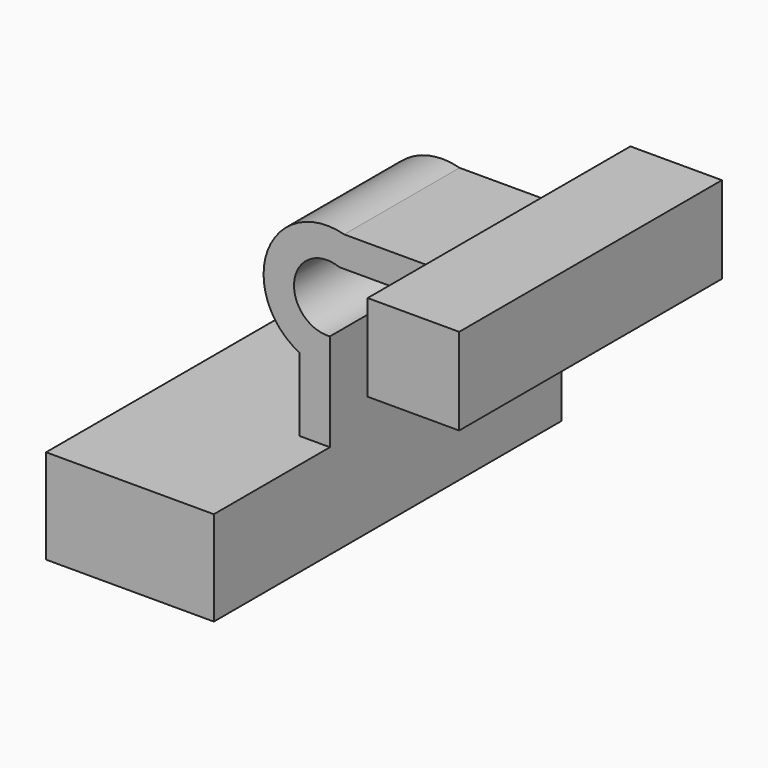
from build123d import *

# Parameters (mm, degrees)
F1_DEPTH = 63.5
F2_DEPTH = 21.082
F3_DEPTH = 48.006


# Not quite as in the source:
# - a feature of the source that left no trace in its solid (it failed there, or was rolled back) is left out


with BuildPart() as f1:
    # F0 (on Front) → F1 (new body, symmetric)
    with BuildSketch(Plane.XZ):
        Polygon((0, -27.6409685612), (0, 0), (-8.890000172, 0), (-49.0482896566, 0), (-49.0482896566, -27.6409685612), align=None)
    extrude(amount=F1_DEPTH, both=True)

    # F0 (on Front) → F2 (join, symmetric)
    with BuildSketch(Plane.XZ):
        with BuildLine():
            Line((-8.890000172, 0), (0, 0))
            Line((0, 0), (0, 28.5326149315))
            ThreePointArc((0, 28.5326149315), (-10.4057051367, 39.6136101279), (2.7482079064, 47.2321221605))
            Line((2.7482079064, 47.2321221605), (32.5638093054, 47.2321221605))
            Line((32.5638093054, 47.2321221605), (32.5638093054, 56.1221223325))
            Line((32.5638093054, 56.1221223325), (4.1557957579, 56.1221223325))
            ThreePointArc((4.1557957579, 56.1221223325), (-18.2071887125, 44.7519974591), (-8.890000172, 21.4588050682))
            Line((-8.890000172, 21.4588050682), (-8.890000172, 0))
        make_face()
    extrude(amount=F2_DEPTH, both=True)

    # F0 (on Front) → F3 (join, symmetric)
    with BuildSketch(Plane.XZ):
        Polygon((32.5638093054, 56.1221223325), (32.5638093054, 47.2321221605), (32.5638093054, 34.5321221605), (59.3218803406, 34.5321221605), (59.3218803406, 59.9321221605), (32.5638093054, 59.9321221605), align=None)
    extrude(amount=F3_DEPTH, both=True)


solid = f1.part
